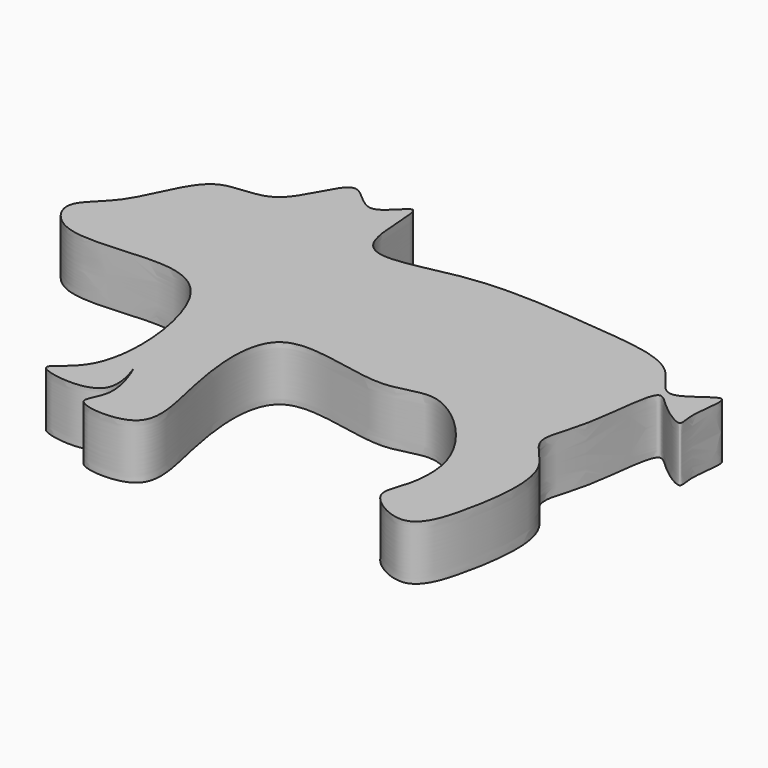
from build123d import *

# Parameters (mm, degrees)
F1_DEPTH = 5


with BuildPart() as f1:
    # F0 (on Top) → F1 (new body)
    with BuildSketch(Plane.XY):
        with BuildLine():
            add(Edge.make_bspline(
                [(-5.7958532125, 41.3069538772), (-1.5023227633, 42.0139265126), (6.4006578907, 41.098491499), (14.9780649484, 40.4499787429), (16.8219474993, 34.8410780305), (21.5227775113, 39.9953598091), (20.1761898121, 34.8604489974), (21.0659279109, 32.702403225), (18.037615758, 34.7438168336), (16.0620539512, 37.1554536358), (15.7990552936, 28.715400599), (13.5953648934, 24.7855032348), (18.2267515341, 21.8877508635), (17.313477333, 13.933857727), (15.4384578213, 8.0311485273), (10.1097938715, 11.1721056819), (11.3779216042, 13.6429470739), (12.2153238793, 19.5963089054), (4.664691376, 27.1361075182), (0.4083011663, 23.6310499935), (-11.7737961921, 28.552865839), (-10.367141144, 16.2253304178), (-7.8195021007, 8.3571237164), (-16.1697731875, 8.9819165124), (-13.1178925431, 11.5354202761), (-16.0144214452, 17.8521108141), (-12.7916984028, 10.3169710238), (-22.3110698072, 11.6764112707), (-15.8040915169, 13.8650612273), (-17.4066633323, 27.8767973034), (-23.7571527111, 30.2438134545), (-32.3780435833, 28.3562042138), (-35.3892455885, 32.8453920526), (-31.1947474588, 35.1412286843), (-29.2463738371, 43.0954505553), (-22.7197529249, 40.9701623777), (-20.6325297336, 49.5763885284), (-17.2906373589, 43.7691361124), (-13.8170789563, 49.8068886834), (-15.3909785175, 38.2864446157), (-9.1850861114, 40.7488828578), (-5.7958532125, 41.3069538772)],
                knots=[0, 0, 0, 0, 0.0404957746, 0.0726168535, 0.0946985699, 0.11607882, 0.1367611125, 0.1505493056, 0.1695951919, 0.1845682399, 0.2140900457, 0.2376438777, 0.260614569, 0.2925811786, 0.3176380176, 0.3406898175, 0.3576060778, 0.3847552199, 0.4185585339, 0.4432601236, 0.477933052, 0.5124585538, 0.5421111852, 0.566485496, 0.5842915413, 0.6064255251, 0.6276892591, 0.6534928256, 0.6736097607, 0.7135477368, 0.741602976, 0.7743085845, 0.7953943665, 0.818004413, 0.8479504847, 0.873246189, 0.8999469087, 0.9208336041, 0.9402177736, 0.9680333904, 1, 1, 1, 1], degree=3))
        make_face()
    extrude(amount=F1_DEPTH)


solid = f1.part
